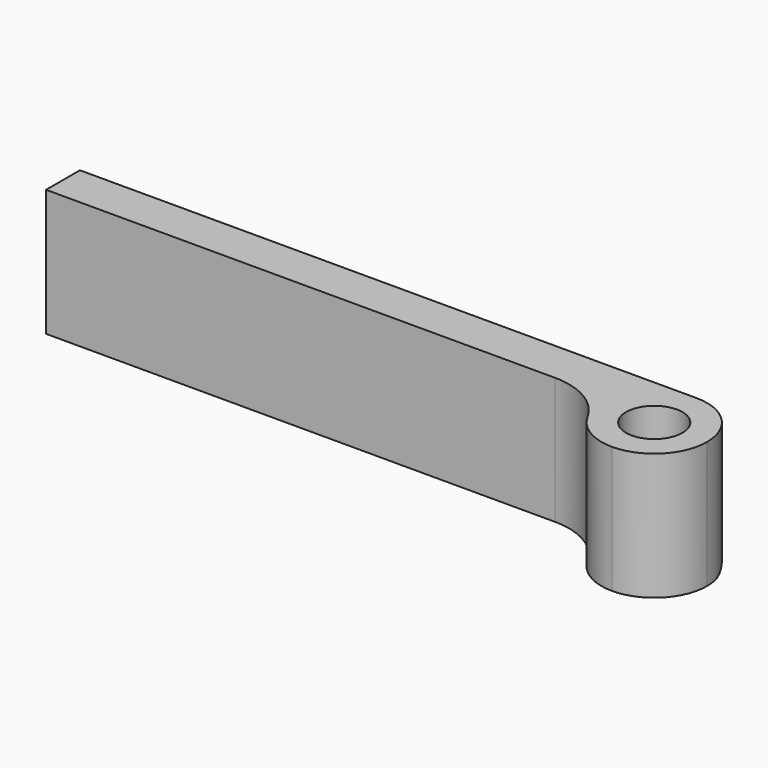
from build123d import *

# Parameters (mm, degrees)
F0_R        = 10
F0_W        = 200
F0_H        = 15
F1_DEPTH    = 45
F2_T1_DEPTH = 138.75
F3_R        = 25
F4_T1_DEPTH = 293.75


# Not quite as in the source:
# - a fillet or chamfer that OpenCascade refuses, or shapes differently, is made with other operations: its cross-section is extruded or revolved along the edge and cut away or added


with BuildPart() as f1:
    # F0 (on Top) → F1 (new body)
    with BuildSketch(Plane.XY):
        Polygon((118.75, -18.75), (118.75, 18.75), (81.25, 18.75), (81.25, 3.75), (81.25, -18.75), align=None)
        with Locations((100, 0)):
            Circle(F0_R, mode=Mode.SUBTRACT)
        with Locations((-18.75, 11.25)):
            Rectangle(F0_W, F0_H)
    extrude(amount=F1_DEPTH)

    # F2: fillet of radius 18.75 on 3 edges, made by hand

    # F2_s2 → F2_t1 (cut)
    with BuildSketch(Plane.XY.offset(-46.875)):
        with BuildLine():
            ThreePointArc((118.75, 0), (113.2582521472, 13.2582521472), (100, 18.75))
            Line((100, 18.75), (118.75, 18.75))
            Line((118.75, 18.75), (118.75, 0))
        make_face()
        with BuildLine():
            ThreePointArc((118.75, 0), (113.2582521472, -13.2582521472), (100, -18.75))
            Line((100, -18.75), (118.75, -18.75))
            Line((118.75, -18.75), (118.75, 0))
        make_face()
        with BuildLine():
            ThreePointArc((81.25, 0), (86.7417478528, -13.2582521472), (100, -18.75))
            Line((100, -18.75), (81.25, -18.75))
            Line((81.25, -18.75), (81.25, 0))
        make_face()
    extrude(amount=F2_T1_DEPTH, mode=Mode.SUBTRACT)

    # F3
    f3_edges = [f1.edges().sort_by_distance(p)[0] for p in [
        (81.25, 3.75, 22.5),
    ]]
    fillet(f3_edges, radius=F3_R)

    # F4: fillet of radius 15 on 2 edges, made by hand

    # F4_s2 → F4_t1 (cut)
    with BuildSketch(Plane.YZ.offset(-156.25)):
        with BuildLine():
            ThreePointArc((3.75, 0), (14.3566017178, 4.3933982822), (18.75, 15))
            Line((18.75, 15), (18.75, 0))
            Line((18.75, 0), (3.75, 0))
        make_face()
    extrude(amount=F4_T1_DEPTH, mode=Mode.SUBTRACT)


solid = f1.part
